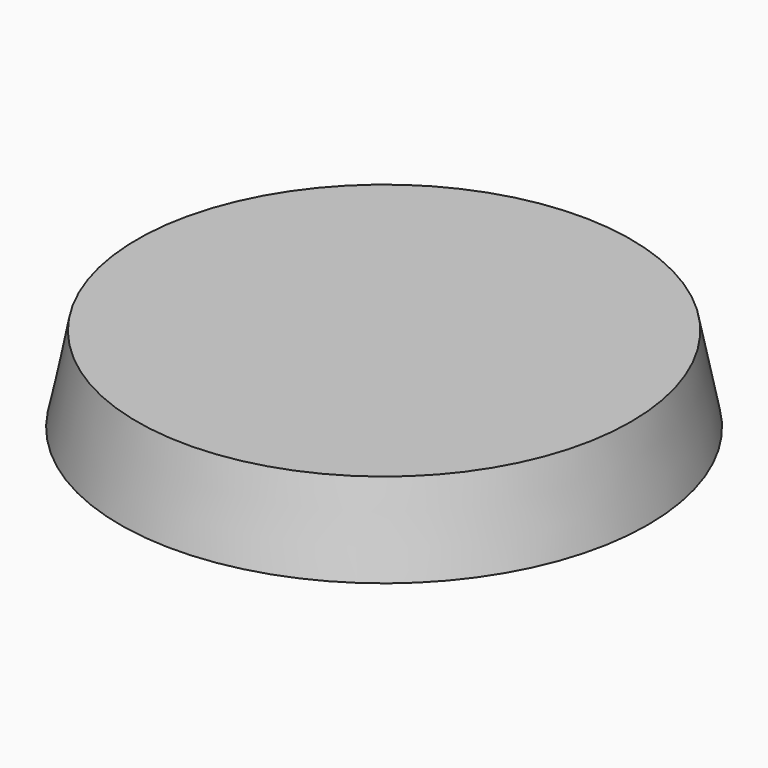
from build123d import *

# Parameters (mm, degrees)
F0_R     = 15.5
F1_DEPTH = 5
F2_SIZE2 = 4.99999
F2_SIZE  = 0.99999
F3_W     = 10
F3_H     = 2
F4_DEPTH = 2


# Not quite as in the source:
# - a fillet or chamfer is up to 0.001 mm smaller than in the source, because OpenCascade refuses the exact size


with BuildPart() as f1:
    # F0 (on Top) → F1 (new body)
    with BuildSketch(Plane.XY):
        Circle(F0_R)
    extrude(amount=F1_DEPTH)

    # F2 (size 1 and 5 in the source; OpenCascade refuses exactly that, so slightly less here)
    f2_edges = [f1.edges().sort_by_distance(p)[0] for p in [
        (-15.5, 0, 5),
    ]]
    f2_side = f1.faces().sort_by_distance((0, 0, 5))[0]
    chamfer(f2_edges, length=F2_SIZE, length2=F2_SIZE2, reference=f2_side)

    # F3 (on face) → F4 (cut)
    with BuildSketch(Plane(origin=(0, 0, 0), x_dir=(1, 0, 0), z_dir=(0, 0, -1))):
        with Locations((0.2559603993, -0.1766888017)):
            Rectangle(F3_W, F3_H)
    extrude(amount=-F4_DEPTH, mode=Mode.SUBTRACT)


solid = f1.part
